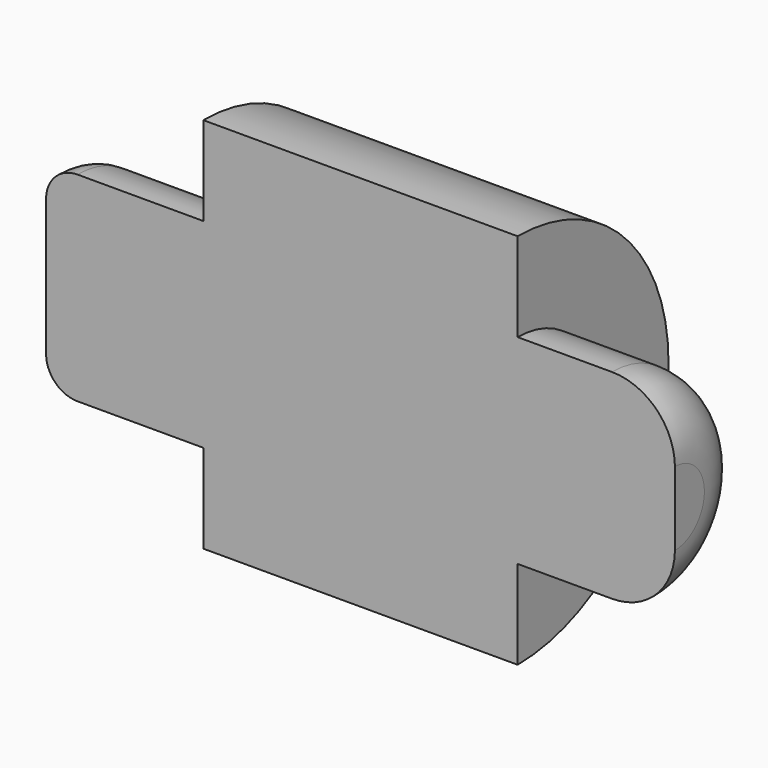
from build123d import *

# Parameters (mm, degrees)
F1_ANGLE_BACK = 90
F1_ANGLE      = 180
F2_T          = 1
F2_T4_ANGLE   = 180.000000001
F2_T6_ANGLE   = 180.000000001
F3_R          = 1
F4_R          = 0.5


# Not quite as in the source:
# - a feature of the source that left no trace in its solid (it failed there, or was rolled back) is left out
# - a shell that OpenCascade refuses in one call is made with other operations: the cavity is built on its own and cut out


with BuildPart() as f1:
    # F0 (on Top) → F1 (revolve)
    with BuildSketch(Plane.XY, mode=Mode.PRIVATE) as f1_sk:
        Polygon((-2.5, 1.5875), (-5, 1.5875), (-5, 0), (5, 0), (5, 1.5875), (2.5, 1.5875), (2.5, 3), (-2.5, 3), align=None)
    revolve(f1_sk.sketch.rotate(Axis((0.2477309544, 0, 0), (1, 0, 0)), -F1_ANGLE_BACK), axis=Axis((0.2477309544, 0, 0), (1, 0, 0)), revolution_arc=F1_ANGLE)

    # F2: shell of thickness 1, made by hand


with BuildPart() as f2_core1:
    # F2_t2: copy of F1
    add(f1.part)

    # the walls: a layer under each face that stays
    f2_faces = [f2_core1.faces().sort_by_distance(p)[0] for p in [
        (-3.75, 1.5875, 0),
        (0, 0, 0),
        (3.75, 1.5875, 0),
        (2.5, 0.5, -2),
        (0, 3, 0),
        (-2.5, 0.5, 2),
    ]]
    thicken(f2_faces, amount=-F2_T, mode=Mode.SUBTRACT)

    # F2_s3 → F2_t4 (revolve, cut)
    with BuildSketch(Plane.XZ):
        Polygon((-2.51, -1.5975), (-2.5, -0.5875), (-1.5, -0.5875), (-1.5, -1.5875), align=None)
    revolve(axis=Axis((-2.5, 0, 0), (1, 0, 0)), revolution_arc=F2_T4_ANGLE, mode=Mode.SUBTRACT)

    # F2_s5 → F2_t6 (revolve, cut)
    with BuildSketch(Plane.XZ):
        Polygon((2.51, -1.5975), (2.5, -0.5875), (1.5, -0.5875), (1.5, -1.5875), align=None)
    revolve(axis=Axis((2.5, 0, 0), (1, 0, 0)), revolution_arc=F2_T6_ANGLE, mode=Mode.SUBTRACT)


with BuildPart() as f1_1:
    add(f1.part)

    # what is left inside the walls is the cavity
    f2_cavity = [f2_core1.part.solids().sort_by_distance(p)[0] for p in [
        (0.5, 1.99, 0),
    ]]
    add(f2_cavity, mode=Mode.SUBTRACT)

    # F3
    f3_edges = [f1_1.edges().sort_by_distance(p)[0] for p in [
        (5, 1.5875, 0),
    ]]
    fillet(f3_edges, radius=F3_R)

    # F4
    f4_edges = [f1_1.edges().sort_by_distance(p)[0] for p in [
        (-5, 1.5875, 0),
    ]]
    fillet(f4_edges, radius=F4_R)


solid = f1_1.part
